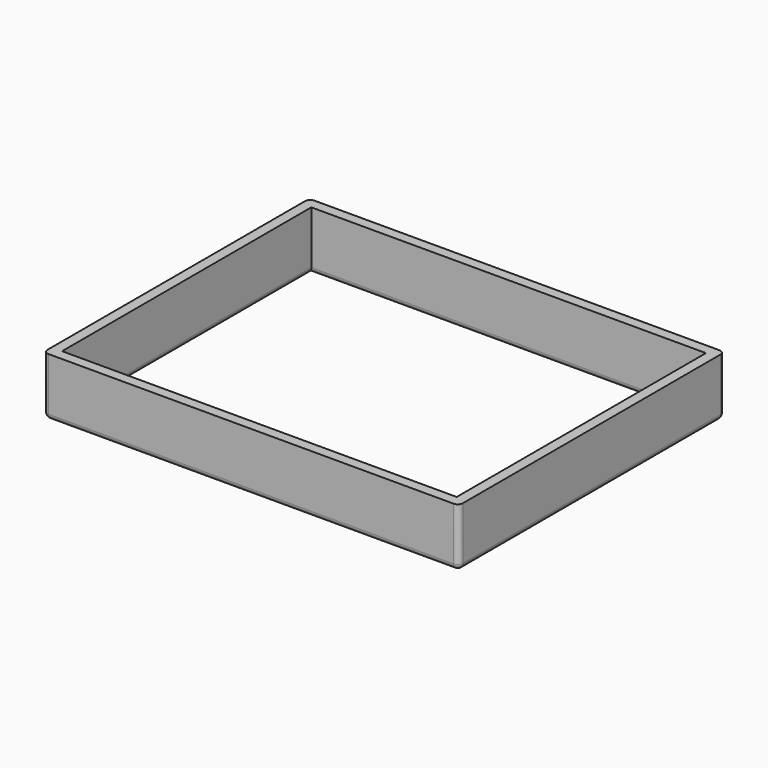
from build123d import *

# Parameters (mm, degrees)
F0_W     = 40
F0_H     = 32
F0_W_2   = 38
F0_H_2   = 30
F1_DEPTH = 5.6
F2_R     = 0.49999


# Not quite as in the source:
# - a fillet or chamfer is up to 0.001 mm smaller than in the source, because OpenCascade refuses the exact size


with BuildPart() as f1:
    # F0 (on Top) → F1 (new body)
    with BuildSketch(Plane.XY):
        Rectangle(F0_W, F0_H)
        Rectangle(F0_W_2, F0_H_2, mode=Mode.SUBTRACT)
    extrude(amount=F1_DEPTH)

    # F2 (radius 0.5 in the source; OpenCascade refuses exactly that, so slightly less here)
    f2_edges = [f1.edges().sort_by_distance(p)[0] for p in [
        (0, 16, 0),
        (-20, 0, 0),
        (0, -16, 0),
        (20, 0, 0),
        (0, 15, 0),
        (19, 0, 0),
        (0, -15, 0),
        (-19, 0, 0),
        (-20, -16, 2.8),
        (20, -16, 2.8),
        (-20, 16, 2.8),
        (20, 16, 2.8),
    ]]
    fillet(f2_edges, radius=F2_R)


solid = f1.part
